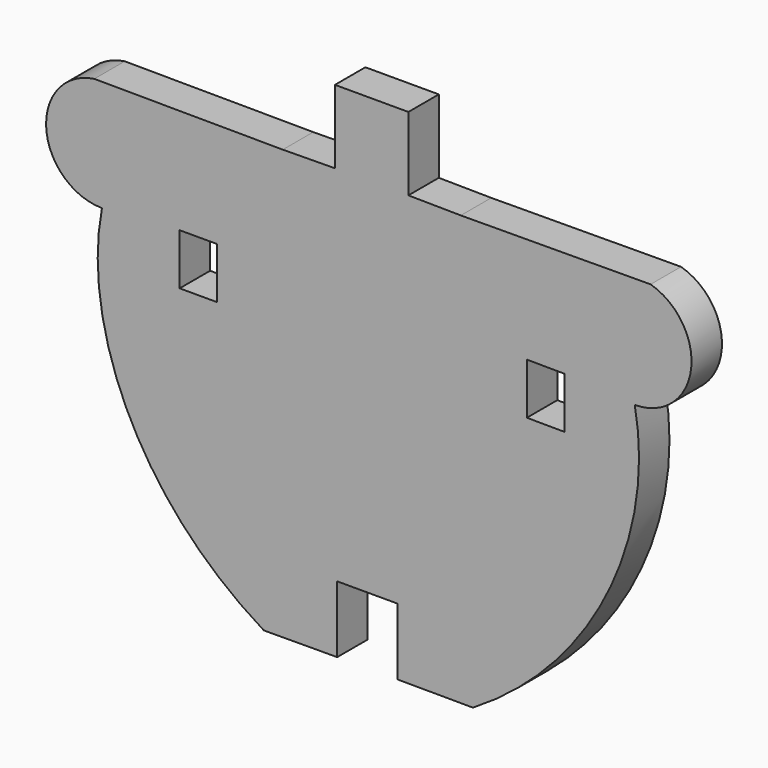
from build123d import *

# Parameters (mm, degrees)
F0_W     = 4.2672
F0_H     = 5.842
F1_DEPTH = 4.3434


with BuildPart() as f1:
    # F0 (on Front) → F1 (new body)
    with BuildSketch(Plane.XZ):
        with BuildLine():
            Line((2.1634316072, 10.8543494716), (-19.3501866255, 10.9726172321))
            ThreePointArc((-19.3501866255, 10.9726172321), (-24.8410026739, 4.2145660489), (-18.4759762851, -1.7273827679))
            add(Edge.make_bspline(
                [(-18.4759762851, -1.7273827679), (-20.8852616932, -14.0894673655), (-14.3136853987, -29.476307077), (0, -38.1591799864)],
                knots=[0, 0, 0, 0, 0.1710209887, 0.1710209887, 0.1710209887, 0.1710209887], degree=3))
            Line((0, -38.1591799864), (8.3743836731, -38.1230656058))
            Line((8.3743836731, -38.1230656058), (8.3743836731, -30.5030656058))
            Line((8.3743836731, -30.5030656058), (12.2675002734, -30.5030656058))
            Line((12.2675002734, -30.5030656058), (15.2323836731, -30.5030656058))
            Line((15.2323836731, -30.5030656058), (15.2323836731, -38.1230656058))
            Line((15.2323836731, -38.1230656058), (23.8656476492, -38.1591799864))
            add(Edge.make_bspline(
                [(42.3416239343, -1.7273827679), (44.7509093424, -14.0894673655), (38.1793330479, -29.476307077), (23.8656476492, -38.1591799864)],
                knots=[0, 0, 0, 0, 0.1710209887, 0.1710209887, 0.1710209887, 0.1710209887], degree=3))
            ThreePointArc((42.3416239343, -1.7273827679), (48.7556622303, 3.8381273274), (44.1498133745, 10.9726172321))
            Line((44.1498133745, 10.9726172321), (22.4834316072, 10.8543494716))
            Line((22.4834316072, 10.8543494716), (16.4287500314, 10.9232757241))
            Line((16.4287500314, 10.9232757241), (16.4984082512, 10.9232757241))
            Line((16.4984082512, 10.9232757241), (16.4984082512, 19.3052757241))
            Line((16.4984082512, 19.3052757241), (8.1164082512, 19.3052757241))
            Line((8.1164082512, 19.3052757241), (8.1164082512, 10.9232757241))
            Line((8.1164082512, 10.9232757241), (8.294825498, 10.9232757241))
            Line((8.294825498, 10.9232757241), (2.1634316072, 10.8543494716))
        make_face()
        with Locations((-7.4751781712, -3.9884169885)):
            Rectangle(F0_W, F0_H, mode=Mode.SUBTRACT)
        Polygon((30.0267527077, -7.0222468014), (30.0640258865, -1.180365708), (34.331139033, -1.2075913342), (34.2938658543, -7.0494724276), align=None, mode=Mode.SUBTRACT)
    extrude(amount=F1_DEPTH)


solid = f1.part
